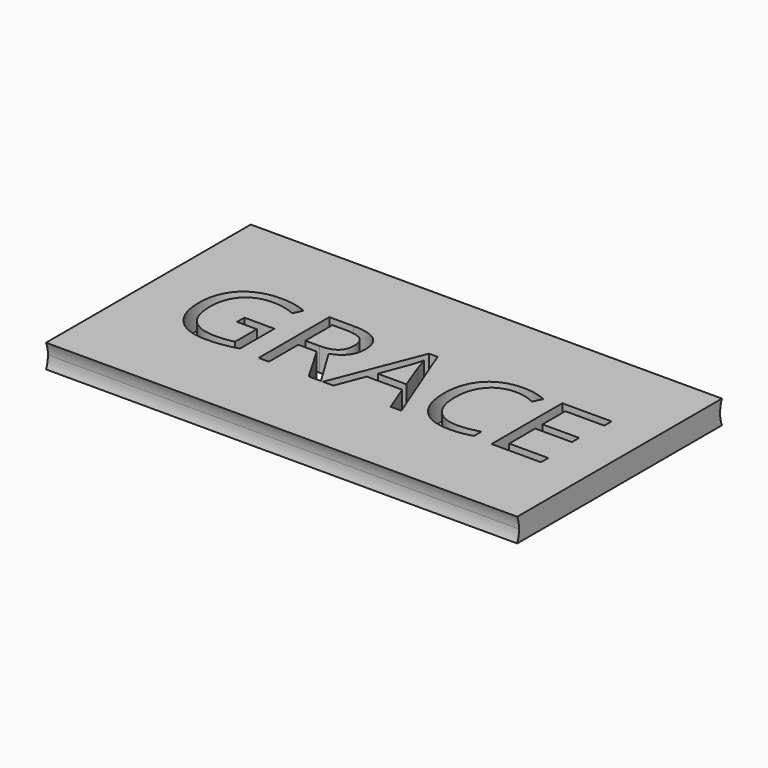
from build123d import *

# Parameters (mm, degrees)
F1_DEPTH     = 38.1
F2_TEXT_SIZE = 10.0133050806
F3_DEPTH     = 25.4


# Not quite as in the source:
# - Text() gives the source's letters only with a copy of the font that has no kerning and outlines rounded to 1/6400 em; it was checked with that copy


with BuildPart() as f1:
    # F0 (on Right) → F1 (new body)
    with BuildSketch(Plane.YZ):
        with BuildLine():
            Line((0, 0), (-12.7413007861, 0))
            ThreePointArc((-12.7413007861, 0), (-12.7880706252, -0.4851838466), (-12.9266577664, -0.9525))
            Line((-12.9266577664, -0.9525), (0, -0.9525))
            Line((0, -0.9525), (0, 0))
        make_face()
        with BuildLine():
            ThreePointArc((-12.9266577664, 0.9525), (-12.7880706252, 0.4851838466), (-12.7413007861, 0))
            Line((-12.7413007861, 0), (0, 0))
            Line((0, 0), (0, 0.9525))
            Line((0, 0.9525), (-12.9266577664, 0.9525))
        make_face()
        with BuildLine():
            Line((7.5786992139, 0), (0, 0))
            Line((0, 0), (0, -0.9525))
            Line((0, -0.9525), (7.7640561943, -0.9525))
            ThreePointArc((7.7640561943, -0.9525), (7.6254690531, -0.4851838466), (7.5786992139, 0))
        make_face()
        with BuildLine():
            Line((0, 0.9525), (0, 0))
            Line((0, 0), (7.5786992139, 0))
            ThreePointArc((7.5786992139, 0), (7.6254690531, 0.4851838466), (7.7640561943, 0.9525))
            Line((7.7640561943, 0.9525), (0, 0.9525))
        make_face()
    extrude(amount=F1_DEPTH)

    # F2 (on face) → F3 (cut)
    with BuildSketch(Plane.XY.offset(0.9525)):
        with Locations((3.5097690616, -6.1753155836)):
            Text('GRACE', F2_TEXT_SIZE, font='Open Sans', text_align=(TextAlign.LEFT, TextAlign.BOTTOM))
    extrude(amount=-F3_DEPTH, mode=Mode.SUBTRACT)


solid = f1.part
